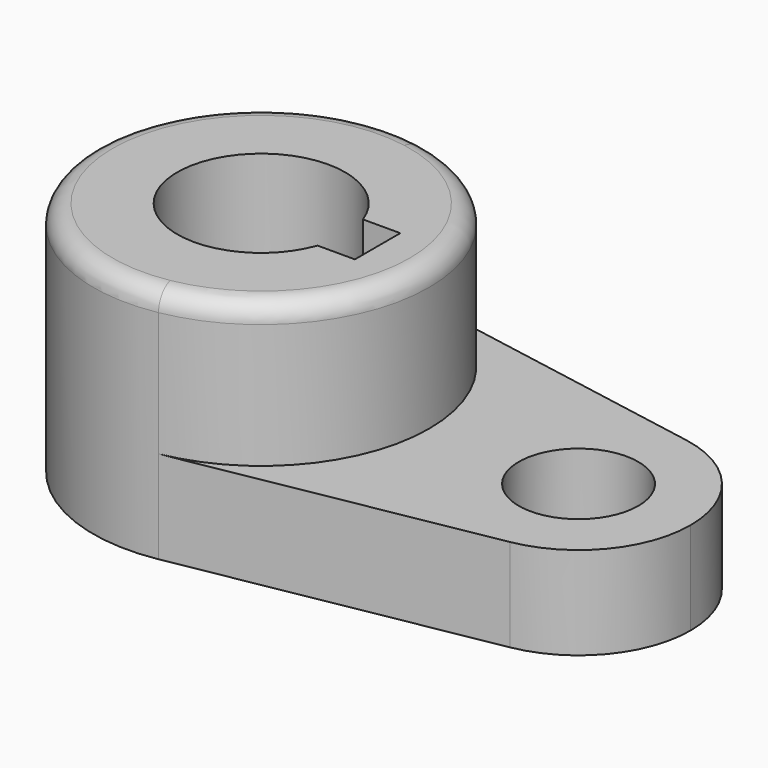
from build123d import *

# Parameters (mm, degrees)
F1_DEPTH = 40.2336
F0_R     = 10.16
F2_DEPTH = 15.7734
F3_R     = 3.302


# Not quite as in the source:
# - a feature names something its author has since deleted; it is built from what else it names


with BuildPart() as f1:
    # F0 (on Top) → F1 (new body)
    with BuildSketch(Plane.XY):
        with BuildLine():
            ThreePointArc((5.0426470588, -28.1265414802), (21.9160245563, -18.3362616868), (28.575, 0))
            ThreePointArc((28.575, 0), (21.9160245563, 18.3362616868), (5.0426470588, 28.1265414802))
            ThreePointArc((5.0426470588, 28.1265414802), (-28.575, 0), (5.0426470588, -28.1265414802))
        make_face()
        with BuildLine():
            ThreePointArc((13.4477648793, -4.826), (-14.2875, 0), (13.4477648793, 4.826))
            Line((13.4477648793, 4.826), (19.7977648793, 4.826))
            Line((19.7977648793, 4.826), (19.7977648793, -4.826))
            Line((19.7977648793, -4.826), (13.4477648793, -4.826))
        make_face(mode=Mode.SUBTRACT)
    extrude(amount=F1_DEPTH)

    # F0 (on Top) → F2 (join)
    with BuildSketch(Plane.XY):
        with BuildLine():
            ThreePointArc((5.0426470588, 28.1265414802), (21.9160245563, 18.3362616868), (28.575, 0))
            ThreePointArc((28.575, 0), (21.9160245563, -18.3362616868), (5.0426470588, -28.1265414802))
            Line((5.0426470588, -28.1265414802), (57.3367647059, -18.7510276535))
            ThreePointArc((57.3367647059, -18.7510276535), (34.925, 0), (57.3367647059, 18.7510276535))
            Line((57.3367647059, 18.7510276535), (5.0426470588, 28.1265414802))
        make_face()
        with BuildLine():
            ThreePointArc((73.025, 0), (68.5856830375, 12.2241744579), (57.3367647059, 18.7510276535))
            ThreePointArc((57.3367647059, 18.7510276535), (34.925, 0), (57.3367647059, -18.7510276535))
            ThreePointArc((57.3367647059, -18.7510276535), (68.5856830375, -12.2241744579), (73.025, 0))
        make_face()
        with Locations((53.975, 0)):
            Circle(F0_R, mode=Mode.SUBTRACT)
    extrude(amount=F2_DEPTH)

    # F3
    f3_edges = [f1.edges().sort_by_distance(p)[0] for p in [
        (-5.042647, 28.126541, 40.2336),
    ]]
    fillet(f3_edges, radius=F3_R)


solid = f1.part
